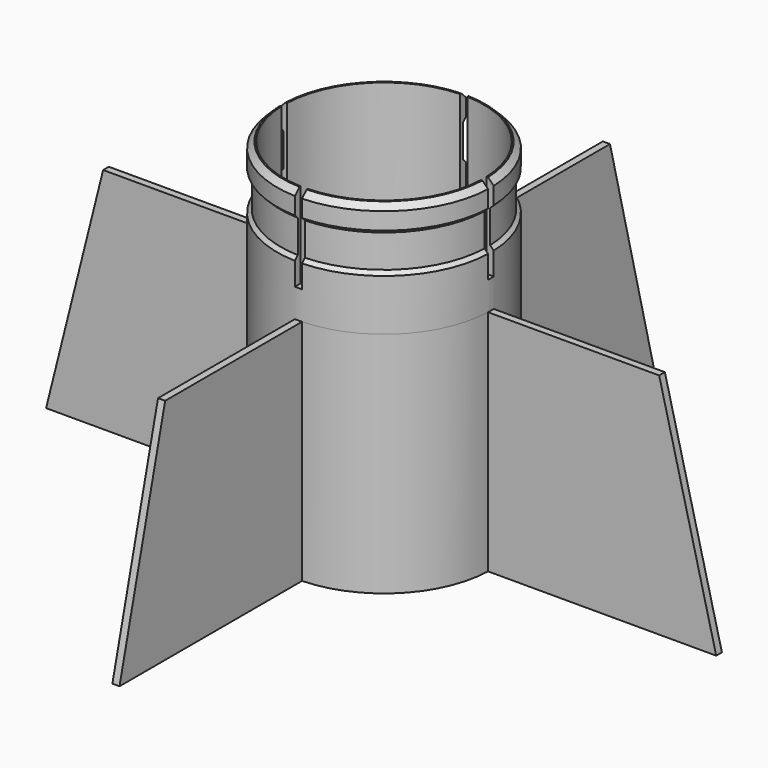
from build123d import *

# Parameters (mm, degrees)
F0_R         = 44.45
F1_DEPTH     = 76.2
F2_R         = 47.625
F2_R_2       = 44.45
F3_DEPTH     = 127
F4_W         = 3.175
F4_H         = 46.0375
F4_H_2       = 3.175
F4_W_2       = 46.0375
F5_DEPTH     = 38.1
F6_W         = 1.5875
F6_H         = 12.7
F8_T2_ANGLE  = 101.902331204
F8_T6_ANGLE  = 101.902331204
F8_S7_R      = 46.0375
F8_T8_DEPTH  = 39
F8_T12_ANGLE = 101.902331204
F8_S13_R     = 46.0375
F8_T14_DEPTH = 39
F8_T18_ANGLE = 101.902331204
F8_S19_R     = 46.0375
F8_T20_DEPTH = 39
F8_T24_ANGLE = 101.902331204
F8_S25_R     = 46.0375
F8_T26_DEPTH = 39
F8_T28_ANGLE = 101.902331204
F8_T32_ANGLE = 101.902331204
F8_S33_R     = 46.0375
F8_T34_DEPTH = 39
F8_T36_ANGLE = 101.902331204
F8_T40_ANGLE = 101.902331204
F8_S41_R     = 46.0375
F8_T42_DEPTH = 39
F8_T44_ANGLE = 101.902331204
F8_T48_ANGLE = 101.902331204
F8_S49_R     = 46.0375
F8_T50_DEPTH = 39
F8_T54_ANGLE = 101.902331204
F8_S55_R     = 46.0375
F8_T56_DEPTH = 39
F9_DEPTH     = 25.4
F11_DEPTH    = 3.175
F13_DEPTH    = 3.175
F15_DEPTH    = 3.175
F17_DEPTH    = 3.175


# Not quite as in the source:
# - a fillet or chamfer that OpenCascade refuses, or shapes differently, is made with other operations: its cross-section is extruded or revolved along the edge and cut away or added


with BuildPart() as f1:
    # F0 (on Top) → F1 (new body)
    with BuildSketch(Plane.XY):
        with BuildLine():
            Line((101.6, 1.5875), (47.598534313, 1.5875))
            ThreePointArc((47.598534313, 1.5875), (33.675960454, 33.675960454), (1.5875, 47.598534313))
            Line((1.5875, 47.598534313), (1.5875, 101.5875968992))
            Line((1.5875, 101.5875968992), (-1.5875, 101.5875968992))
            Line((-1.5875, 101.5875968992), (-1.5875, 47.598534313))
            ThreePointArc((-1.5875, 47.598534313), (-33.675960454, 33.675960454), (-47.598534313, 1.5875))
            Line((-47.598534313, 1.5875), (-101.6, 1.5875))
            Line((-101.6, 1.5875), (-101.6, -1.5875))
            Line((-101.6, -1.5875), (-47.598534313, -1.5875))
            ThreePointArc((-47.598534313, -1.5875), (-33.675960454, -33.675960454), (-1.5875, -47.598534313))
            Line((-1.5875, -47.598534313), (-1.5875, -101.6))
            Line((-1.5875, -101.6), (1.5875, -101.6))
            Line((1.5875, -101.6), (1.5875, -47.598534313))
            ThreePointArc((1.5875, -47.598534313), (33.675960454, -33.675960454), (47.598534313, -1.5875))
            Line((47.598534313, -1.5875), (101.6, -1.5875))
            Line((101.6, -1.5875), (101.6, 1.5875))
        make_face()
        Circle(F0_R, mode=Mode.SUBTRACT)
    extrude(amount=F1_DEPTH)

    # F2 (on Top) → F3 (join)
    with BuildSketch(Plane.XY):
        Circle(F2_R)
        Circle(F2_R_2, mode=Mode.SUBTRACT)
    extrude(amount=F3_DEPTH)

    # F4 (on face) → F5 (cut)
    with BuildSketch(Plane.XY.offset(127)):
        with Locations((0, 24.60625)):
            Rectangle(F4_W, F4_H)
        Rectangle(F4_W, F4_H_2)
        with Locations((-24.60625, 0)):
            Rectangle(F4_W_2, F4_H_2)
        with Locations((0, -24.60625)):
            Rectangle(F4_W, F4_H)
        with Locations((24.60625, 0)):
            Rectangle(F4_W_2, F4_H_2)
    extrude(amount=-F5_DEPTH, mode=Mode.SUBTRACT)

    # F6 (on Right) → F7 (revolve, cut)
    with BuildSketch(Plane.YZ):
        with Locations((-46.83125, 107.95)):
            Rectangle(F6_W, F6_H)
    revolve(axis=Axis((0, 0, 63.5), (0, 0, 1)), mode=Mode.SUBTRACT)

    # F8: chamfer of 2.54 on 12 edges, made by hand

    # F8_s1 → F8_t2 (revolve, cut)
    with BuildSketch(Plane(origin=(0, 0, 0), x_dir=(0, 0, 1), z_dir=(0.1036807735, 0.9946106259, 0))):
        Polygon((127, -45.085), (124.46, -47.625), (127, -47.625), align=None)
    revolve(axis=Axis((0, 0, 127), (0, 0, 1)), revolution_arc=F8_T2_ANGLE, mode=Mode.SUBTRACT)


with BuildPart() as f8_tool4:
    # F8_s5 → F8_t6 (revolve)
    with BuildSketch(Plane(origin=(0, 0, 0), x_dir=(0, 0, 1), z_dir=(0.1036807735, 0.9946106259, 0))):
        Polygon((116.84, -47.625), (114.3, -45.085), (114.3, -47.625), align=None)
    revolve(axis=Axis((0, 0, 114.3), (0, 0, 1)), revolution_arc=F8_T6_ANGLE)

    # F8_s7 → F8_t8 (cut, symmetric)
    with BuildSketch(Plane.XY.offset(115.6)):
        Circle(F8_S7_R)
    extrude(amount=F8_T8_DEPTH, both=True, mode=Mode.SUBTRACT)


with BuildPart() as f1_1:
    add(f1.part)

    # F8_t3: cut F8_tool4
    add(f8_tool4.part, mode=Mode.SUBTRACT)


with BuildPart() as f8_tool10:
    # F8_s11 → F8_t12 (revolve)
    with BuildSketch(Plane(origin=(0, 0, 0), x_dir=(0, 0, 1), z_dir=(0.1036807735, 0.9946106259, 0))):
        Polygon((99.06, -47.625), (101.6, -45.085), (101.6, -47.625), align=None)
    revolve(axis=Axis((0, 0, 101.6), (0, 0, 1)), revolution_arc=F8_T12_ANGLE)

    # F8_s13 → F8_t14 (cut, symmetric)
    with BuildSketch(Plane.XY.offset(100.3)):
        Circle(F8_S13_R)
    extrude(amount=F8_T14_DEPTH, both=True, mode=Mode.SUBTRACT)


with BuildPart() as f1_2:
    add(f1_1.part)

    # F8_t9: cut F8_tool10
    add(f8_tool10.part, mode=Mode.SUBTRACT)


with BuildPart() as f8_tool16:
    # F8_s17 → F8_t18 (revolve)
    with BuildSketch(Plane(origin=(0, 0, 0), x_dir=(0, 0, 1), z_dir=(-0.9946106259, 0.1036807735, 0))):
        Polygon((99.06, -47.625), (101.6, -45.085), (101.6, -47.625), align=None)
    revolve(axis=Axis((0, 0, 101.6), (0, 0, 1)), revolution_arc=F8_T18_ANGLE)

    # F8_s19 → F8_t20 (cut, symmetric)
    with BuildSketch(Plane.XY.offset(100.3)):
        Circle(F8_S19_R)
    extrude(amount=F8_T20_DEPTH, both=True, mode=Mode.SUBTRACT)


with BuildPart() as f1_3:
    add(f1_2.part)

    # F8_t15: cut F8_tool16
    add(f8_tool16.part, mode=Mode.SUBTRACT)


with BuildPart() as f8_tool22:
    # F8_s23 → F8_t24 (revolve)
    with BuildSketch(Plane(origin=(0, 0, 0), x_dir=(0, 0, 1), z_dir=(-0.9946106259, 0.1036807735, 0))):
        Polygon((116.84, -47.625), (114.3, -45.085), (114.3, -47.625), align=None)
    revolve(axis=Axis((0, 0, 114.3), (0, 0, 1)), revolution_arc=F8_T24_ANGLE)

    # F8_s25 → F8_t26 (cut, symmetric)
    with BuildSketch(Plane.XY.offset(115.6)):
        Circle(F8_S25_R)
    extrude(amount=F8_T26_DEPTH, both=True, mode=Mode.SUBTRACT)


with BuildPart() as f1_4:
    add(f1_3.part)

    # F8_t21: cut F8_tool22
    add(f8_tool22.part, mode=Mode.SUBTRACT)

    # F8_s27 → F8_t28 (revolve, cut)
    with BuildSketch(Plane(origin=(0, 0, 0), x_dir=(0, 0, 1), z_dir=(-0.9946106259, 0.1036807735, 0))):
        Polygon((127, -45.085), (124.46, -47.625), (127, -47.625), align=None)
    revolve(axis=Axis((0, 0, 127), (0, 0, 1)), revolution_arc=F8_T28_ANGLE, mode=Mode.SUBTRACT)


with BuildPart() as f8_tool30:
    # F8_s31 → F8_t32 (revolve)
    with BuildSketch(Plane(origin=(0, 0, 0), x_dir=(0, 0, 1), z_dir=(0.9946106259, -0.1036807735, 0))):
        Polygon((116.84, -47.625), (114.3, -45.085), (114.3, -47.625), align=None)
    revolve(axis=Axis((0, 0, 114.3), (0, 0, 1)), revolution_arc=F8_T32_ANGLE)

    # F8_s33 → F8_t34 (cut, symmetric)
    with BuildSketch(Plane.XY.offset(115.6)):
        Circle(F8_S33_R)
    extrude(amount=F8_T34_DEPTH, both=True, mode=Mode.SUBTRACT)


with BuildPart() as f1_5:
    add(f1_4.part)

    # F8_t29: cut F8_tool30
    add(f8_tool30.part, mode=Mode.SUBTRACT)

    # F8_s35 → F8_t36 (revolve, cut)
    with BuildSketch(Plane(origin=(0, 0, 0), x_dir=(0, 0, 1), z_dir=(0.9946106259, -0.1036807735, 0))):
        Polygon((127, -45.085), (124.46, -47.625), (127, -47.625), align=None)
    revolve(axis=Axis((0, 0, 127), (0, 0, 1)), revolution_arc=F8_T36_ANGLE, mode=Mode.SUBTRACT)


with BuildPart() as f8_tool38:
    # F8_s39 → F8_t40 (revolve)
    with BuildSketch(Plane(origin=(0, 0, 0), x_dir=(0, 0, 1), z_dir=(0.9946106259, -0.1036807735, 0))):
        Polygon((99.06, -47.625), (101.6, -45.085), (101.6, -47.625), align=None)
    revolve(axis=Axis((0, 0, 101.6), (0, 0, 1)), revolution_arc=F8_T40_ANGLE)

    # F8_s41 → F8_t42 (cut, symmetric)
    with BuildSketch(Plane.XY.offset(100.3)):
        Circle(F8_S41_R)
    extrude(amount=F8_T42_DEPTH, both=True, mode=Mode.SUBTRACT)


with BuildPart() as f1_6:
    add(f1_5.part)

    # F8_t37: cut F8_tool38
    add(f8_tool38.part, mode=Mode.SUBTRACT)

    # F8_s43 → F8_t44 (revolve, cut)
    with BuildSketch(Plane(origin=(0, 0, 0), x_dir=(0, 0, 1), z_dir=(-0.1036807735, -0.9946106259, 0))):
        Polygon((127, -45.085), (124.46, -47.625), (127, -47.625), align=None)
    revolve(axis=Axis((0, 0, 127), (0, 0, 1)), revolution_arc=F8_T44_ANGLE, mode=Mode.SUBTRACT)


with BuildPart() as f8_tool46:
    # F8_s47 → F8_t48 (revolve)
    with BuildSketch(Plane(origin=(0, 0, 0), x_dir=(0, 0, 1), z_dir=(-0.1036807735, -0.9946106259, 0))):
        Polygon((116.84, -47.625), (114.3, -45.085), (114.3, -47.625), align=None)
    revolve(axis=Axis((0, 0, 114.3), (0, 0, 1)), revolution_arc=F8_T48_ANGLE)

    # F8_s49 → F8_t50 (cut, symmetric)
    with BuildSketch(Plane.XY.offset(115.6)):
        Circle(F8_S49_R)
    extrude(amount=F8_T50_DEPTH, both=True, mode=Mode.SUBTRACT)


with BuildPart() as f1_7:
    add(f1_6.part)

    # F8_t45: cut F8_tool46
    add(f8_tool46.part, mode=Mode.SUBTRACT)


with BuildPart() as f8_tool52:
    # F8_s53 → F8_t54 (revolve)
    with BuildSketch(Plane(origin=(0, 0, 0), x_dir=(0, 0, 1), z_dir=(-0.1036807735, -0.9946106259, 0))):
        Polygon((99.06, -47.625), (101.6, -45.085), (101.6, -47.625), align=None)
    revolve(axis=Axis((0, 0, 101.6), (0, 0, 1)), revolution_arc=F8_T54_ANGLE)

    # F8_s55 → F8_t56 (cut, symmetric)
    with BuildSketch(Plane.XY.offset(100.3)):
        Circle(F8_S55_R)
    extrude(amount=F8_T56_DEPTH, both=True, mode=Mode.SUBTRACT)


with BuildPart() as f1_8:
    add(f1_7.part)

    # F8_t51: cut F8_tool52
    add(f8_tool52.part, mode=Mode.SUBTRACT)

    # F9 (add): a face of the model
    f9_faces = [f1_8.faces().sort_by_distance(p)[0] for p in [
        (0, -98.7264057431, 0),
    ]]
    extrude(f9_faces, amount=F9_DEPTH)

    # F10 (on face) → F11 (join, through all)
    with BuildSketch(Plane(origin=(0, 1.5875, 0), x_dir=(-1, 0, 0), z_dir=(0, 1, 0))):
        Polygon((123.7956061959, 76.2), (101.6, 76.2), (101.6, -25.4), (149.198534313, -25.4), align=None)
    extrude(amount=-F11_DEPTH)

    # F12 (on face) → F13 (join, through all)
    with BuildSketch(Plane.YZ.offset(1.5875)):
        Polygon((101.5875968992, 76.2), (101.5875968992, -25.4), (149.198534313, -25.4), (123.798534313, 76.2), align=None)
    extrude(amount=-F13_DEPTH)

    # F14 (on face) → F15 (join, through all)
    with BuildSketch(Plane.XZ.offset(1.5875)):
        Polygon((123.798534313, 76.2), (101.6, 76.2), (101.6, -25.4), (149.198534313, -25.4), align=None)
    extrude(amount=-F15_DEPTH)

    # F16 (on face) → F17 (join, through all)
    with BuildSketch(Plane(origin=(-1.5875, 0, 0), x_dir=(0, -1, 0), z_dir=(-1, 0, 0))):
        Polygon((123.798534313, 76.2), (101.6, 76.2), (101.6, -25.4), (149.198534313, -25.4), align=None)
    extrude(amount=-F17_DEPTH)


solid = f1_8.part
